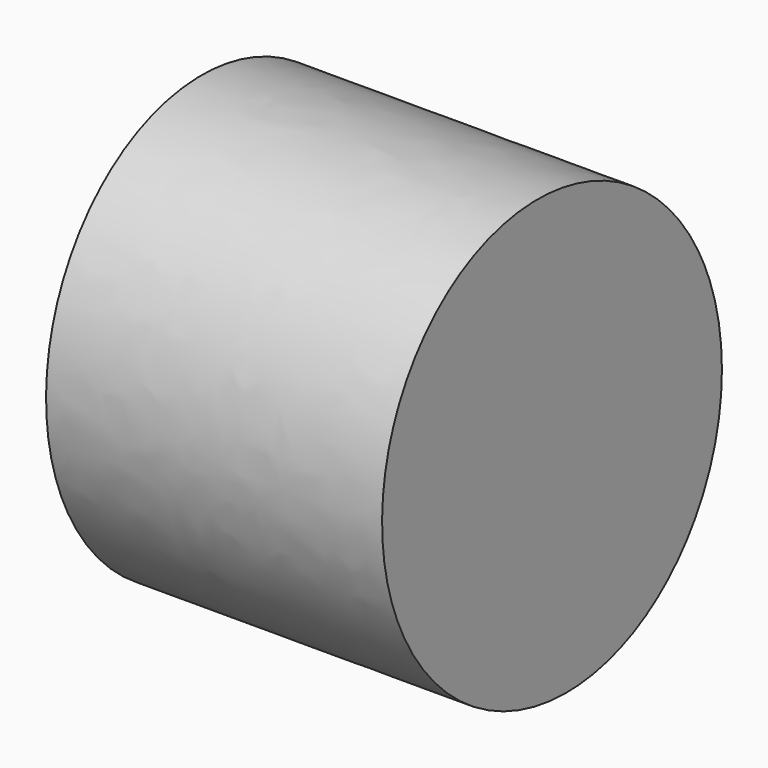
from build123d import *

# Parameters (mm, degrees)
F3_DEPTH = 100


# Not quite as in the source:
# - the program builds the solid bodies; features that only make, move or delete a surface that nothing else refers to are left out


with BuildPart() as f3:
    # F2 (on Right) → F3 (new body)
    with BuildSketch(Plane.YZ):
        with BuildLine():
            add(Edge.make_bspline(
                [(112.8674000502, 29.2646028101), (56.761737081, 133.3254540352), (3.3976673646, 37.3981242075), (-49.9664023519, -58.5292056203), (59.5033303338, -66.6627270176), (168.9730630194, -74.7962484149), (112.8674000502, 29.2646028101)],
                knots=[4.7123889804, 4.7123889804, 4.7123889804, 6.8067840828, 6.8067840828, 8.9011791852, 8.9011791852, 10.9955742876, 10.9955742876, 10.9955742876], degree=2, weights=[1, 0.5, 1, 0.5, 1, 0.5, 1]))
        make_face()
    extrude(amount=F3_DEPTH)


solid = f3.part
